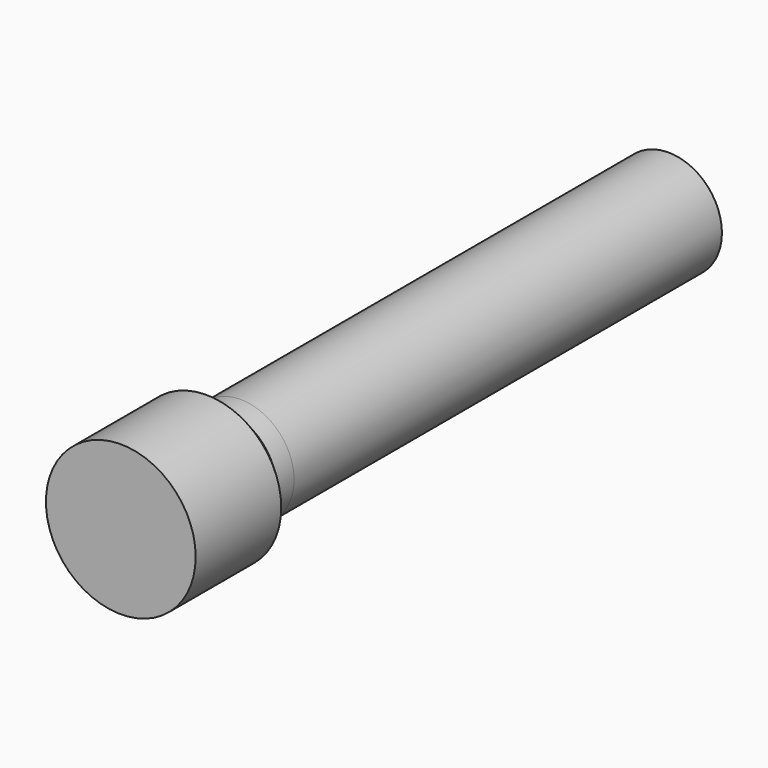
from build123d import *

# Parameters (mm, degrees)
F0_R        = 2.5
F1_DEPTH    = 25
F2_R        = 3.5
F2_R_2      = 2.5
F3_DEPTH    = 7
F4_S5_R     = 2.5
F4_T6_DEPTH = 7


# Not quite as in the source:
# - a fillet or chamfer that OpenCascade refuses, or shapes differently, is made with other operations: its cross-section is extruded or revolved along the edge and cut away or added


with BuildPart() as f1:
    # F0 (on Front) → F1 (new body)
    with BuildSketch(Plane.XZ):
        Circle(F0_R)
    extrude(amount=F1_DEPTH)

    # F2 (on face) → F3 (join)
    with BuildSketch(Plane.XZ.offset(25)):
        Circle(F2_R)
        Circle(F2_R_2, mode=Mode.SUBTRACT)
        Circle(F2_R_2)
    extrude(amount=F3_DEPTH)

    # F4: chamfer of 2 on 1 edges, made by hand


with BuildPart() as f4_tool2:
    # F4_s3 → F4_t4 (revolve)
    with BuildSketch(Plane.XY):
        Polygon((3.5, -27), (1.5, -25), (3.5, -25), align=None)
    revolve(axis=Axis((0, -25, 0), (0, -1, 0)))

    # F4_s5 → F4_t6 (cut, symmetric)
    with BuildSketch(Plane.XZ.offset(26)):
        Circle(F4_S5_R)
    extrude(amount=F4_T6_DEPTH, both=True, mode=Mode.SUBTRACT)


with BuildPart() as f1_1:
    add(f1.part)

    # F4_t1: cut F4_tool2
    add(f4_tool2.part, mode=Mode.SUBTRACT)


solid = f1_1.part
